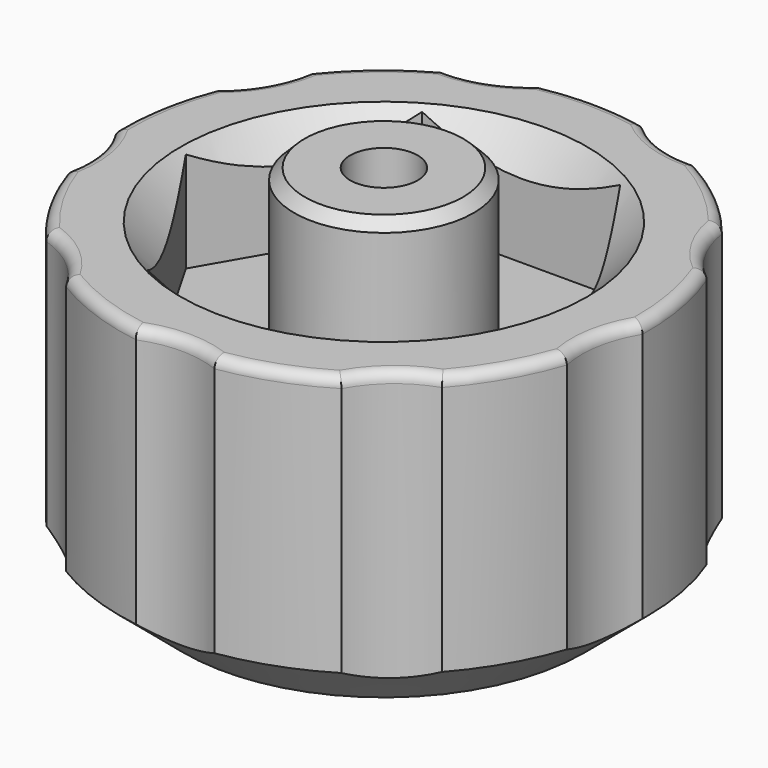
from build123d import *

# Parameters (mm, degrees)
F2_R         = 10
F3_DEPTH     = 30.001
F4_R         = 1
F5_T3_ANGLE  = 72.4183645551
F5_T6_ANGLE  = 34.3109861798
F5_T9_ANGLE  = 34.3109861798
F5_T12_ANGLE = 72.4183645551
F5_T15_ANGLE = 34.3109861798
F5_T18_ANGLE = 72.4183645551
F5_T21_ANGLE = 34.3109861799
F5_T24_ANGLE = 72.4183645551
F5_T27_ANGLE = 34.3109861798
F5_T30_ANGLE = 72.4183645551
F5_T33_ANGLE = 34.3109861799
F5_T36_ANGLE = 72.4183645551
F5_T39_ANGLE = 34.3109861799
F5_T42_ANGLE = 72.4183645551
F5_T45_ANGLE = 34.3109861799
F5_T48_ANGLE = 72.4183645551
F5_T51_ANGLE = 34.3109861798
F5_T54_ANGLE = 72.4183645551
F6_R         = 8.5
F7_DEPTH     = 10


# Not quite as in the source:
# - a fillet or chamfer that OpenCascade refuses, or shapes differently, is made with other operations: its cross-section is extruded or revolved along the edge and cut away or added


with BuildPart() as f1:
    # F0 (on Front) → F1 (revolve)
    with BuildSketch(Plane.XZ):
        Polygon((8, 8), (8.6999093082, 0), (18.6999093082, 0), (25, 5.2864037759), (25, 30), (19.25, 30), (16.25, 27), (16.25, 20), (8.5, 20), (8.5, 33.5), (7.5, 34.5), (3.2, 34.5), (3.2, 8), align=None)
    revolve(axis=Axis((0, 0, 15.2192509614), (0, 0, 1)))

    # F2 (on face) → F3 (cut, through all)
    with BuildSketch(Plane.XY.offset(30)):
        with Locations((11.6286848731, 31.9495491067)):
            Circle(F2_R)
        with Locations((-11.6286848731, 31.9495491067)):
            Circle(F2_R)
        with Locations((-29.4448637287, 17)):
            Circle(F2_R)
        with Locations((-33.4834636024, -5.9040380407)):
            Circle(F2_R)
        with Locations((-21.8547787293, -26.045511066)):
            Circle(F2_R)
        with Locations((0, -34)):
            Circle(F2_R)
        with Locations((21.8547787293, -26.045511066)):
            Circle(F2_R)
        with Locations((33.4834636024, -5.9040380407)):
            Circle(F2_R)
        with Locations((29.4448637287, 17)):
            Circle(F2_R)
    extrude(amount=-F3_DEPTH, mode=Mode.SUBTRACT)

    # F4
    f4_edges = [f1.edges().sort_by_distance(p)[0] for p in [
        (-8.699909, 0, 0),
        (-18.699909, 0, 0),
    ]]
    fillet(f4_edges, radius=F4_R)

    # F5: fillet of radius 1 on 18 edges, made by hand


with BuildPart() as f5_tool1:
    # F5_s2 → F5_t3 (revolve)
    with BuildSketch(Plane(origin=(4.7878159953, -19.5059893322, 0), x_dir=(0, 0, 1), z_dir=(0.2383778196, -0.971172495, 0))):
        with BuildLine():
            ThreePointArc((29, 17.4334321252), (29.7071067812, 17.1405389064), (30, 16.4334321252))
            Line((30, 16.4334321252), (30, 17.4334321252))
            Line((30, 17.4334321252), (29, 17.4334321252))
        make_face()
    revolve(axis=Axis((-21.8547787293, -26.045511066, 30), (0, 0, 1)), revolution_arc=F5_T3_ANGLE)


with BuildPart() as f5_tool4:
    # F5_s5 → F5_t6 (revolve)
    with BuildSketch(Plane(origin=(0, 0, 0), x_dir=(0, 0, 1), z_dir=(-0.7969993255, 0.6039801944, 0))):
        with BuildLine():
            ThreePointArc((29, -25), (29.7071067812, -24.7071067812), (30, -24))
            Line((30, -24), (30, -25))
            Line((30, -25), (29, -25))
        make_face()
    revolve(axis=Axis((0, 0, 30), (0, 0, 1)), revolution_arc=F5_T6_ANGLE)


with BuildPart() as f5_tool7:
    # F5_s8 → F5_t9 (revolve)
    with BuildSketch(Plane(origin=(0, 0, 0), x_dir=(0, 0, 1), z_dir=(-0.222305919, 0.974976963, 0))):
        with BuildLine():
            ThreePointArc((29, -25), (29.7071067812, -24.7071067812), (30, -24))
            Line((30, -24), (30, -25))
            Line((30, -25), (29, -25))
        make_face()
    revolve(axis=Axis((0, 0, 30), (0, 0, 1)), revolution_arc=F5_T9_ANGLE)


with BuildPart() as f5_tool10:
    # F5_s11 → F5_t12 (revolve)
    with BuildSketch(Plane(origin=(-8.8705284196, -18.0200035347, 0), x_dir=(0, 0, 1), z_dir=(-0.4416496426, -0.897187602, 0))):
        with BuildLine():
            ThreePointArc((29, 17.4334321252), (29.7071067812, 17.1405389064), (30, 16.4334321252))
            Line((30, 16.4334321252), (30, 17.4334321252))
            Line((30, 17.4334321252), (29, 17.4334321252))
        make_face()
    revolve(axis=Axis((-33.4834636024, -5.9040380407, 30), (0, 0, 1)), revolution_arc=F5_T12_ANGLE)


with BuildPart() as f5_tool13:
    # F5_s14 → F5_t15 (revolve)
    with BuildSketch(Plane(origin=(0, 0, 0), x_dir=(0, 0, 1), z_dir=(0.4564068976, 0.889771175, 0))):
        with BuildLine():
            ThreePointArc((29, -25), (29.7071067812, -24.7071067812), (30, -24))
            Line((30, -24), (30, -25))
            Line((30, -25), (29, -25))
        make_face()
    revolve(axis=Axis((0, 0, 30), (0, 0, 1)), revolution_arc=F5_T15_ANGLE)


with BuildPart() as f5_tool16:
    # F5_s17 → F5_t18 (revolve)
    with BuildSketch(Plane(origin=(-18.378254002, -8.1022578133, 0), x_dir=(0, 0, 1), z_dir=(-0.9150243287, -0.4033986588, 0))):
        with BuildLine():
            ThreePointArc((29, 17.4334321252), (29.7071067812, 17.1405389064), (30, 16.4334321252))
            Line((30, 16.4334321252), (30, 17.4334321252))
            Line((30, 17.4334321252), (29, 17.4334321252))
        make_face()
    revolve(axis=Axis((-29.4448637287, 17, 30), (0, 0, 1)), revolution_arc=F5_T18_ANGLE)


with BuildPart() as f5_tool19:
    # F5_s20 → F5_t21 (revolve)
    with BuildSketch(Plane(origin=(0, 0, 0), x_dir=(0, 0, 1), z_dir=(0.9215618544, 0.3882315655, 0))):
        with BuildLine():
            ThreePointArc((29, -25), (29.7071067812, -24.7071067812), (30, -24))
            Line((30, -24), (30, -25))
            Line((30, -25), (29, -25))
        make_face()
    revolve(axis=Axis((0, 0, 30), (0, 0, 1)), revolution_arc=F5_T21_ANGLE)


with BuildPart() as f5_tool22:
    # F5_s23 → F5_t24 (revolve)
    with BuildSketch(Plane(origin=(-19.2865902853, 5.6066243856, 0), x_dir=(0, 0, 1), z_dir=(-0.960248962, 0.2791450001, 0))):
        with BuildLine():
            ThreePointArc((29, 17.4334321252), (29.7071067812, 17.1405389064), (30, 16.4334321252))
            Line((30, 16.4334321252), (30, 17.4334321252))
            Line((30, 17.4334321252), (29, 17.4334321252))
        make_face()
    revolve(axis=Axis((-11.6286848731, 31.9495491067, 30), (0, 0, 1)), revolution_arc=F5_T24_ANGLE)


with BuildPart() as f5_tool25:
    # F5_s26 → F5_t27 (revolve)
    with BuildSketch(Plane(origin=(0, 0, 0), x_dir=(0, 0, 1), z_dir=(0.9555077776, -0.2949659082, 0))):
        with BuildLine():
            ThreePointArc((29, -25), (29.7071067812, -24.7071067812), (30, -24))
            Line((30, -24), (30, -25))
            Line((30, -25), (29, -25))
        make_face()
    revolve(axis=Axis((0, 0, 30), (0, 0, 1)), revolution_arc=F5_T27_ANGLE)


with BuildPart() as f5_tool28:
    # F5_s29 → F5_t30 (revolve)
    with BuildSketch(Plane(origin=(-11.1705166275, 16.6921047237, 0), x_dir=(0, 0, 1), z_dir=(-0.556162434, 0.8310736111, 0))):
        with BuildLine():
            ThreePointArc((29, 17.4334321252), (29.7071067812, 17.1405389064), (30, 16.4334321252))
            Line((30, 16.4334321252), (30, 17.4334321252))
            Line((30, 17.4334321252), (29, 17.4334321252))
        make_face()
    revolve(axis=Axis((11.6286848731, 31.9495491067, 30), (0, 0, 1)), revolution_arc=F5_T30_ANGLE)


with BuildPart() as f5_tool31:
    # F5_s32 → F5_t33 (revolve)
    with BuildSketch(Plane(origin=(0, 0, 0), x_dir=(0, 0, 1), z_dir=(0.5423609923, -0.8401455553, 0))):
        with BuildLine():
            ThreePointArc((29, -25), (29.7071067812, -24.7071067812), (30, -24))
            Line((30, -24), (30, -25))
            Line((30, -25), (29, -25))
        make_face()
    revolve(axis=Axis((0, 0, 30), (0, 0, 1)), revolution_arc=F5_T33_ANGLE)


with BuildPart() as f5_tool34:
    # F5_s35 → F5_t36 (revolve)
    with BuildSketch(Plane(origin=(2.1723659067, 19.9671637495, 0), x_dir=(0, 0, 1), z_dir=(0.1081586779, 0.9941336431, 0))):
        with BuildLine():
            ThreePointArc((29, 17.4334321252), (29.7071067812, 17.1405389064), (30, 16.4334321252))
            Line((30, 16.4334321252), (30, 17.4334321252))
            Line((30, 17.4334321252), (29, 17.4334321252))
        make_face()
    revolve(axis=Axis((29.4448637287, 17, 30), (0, 0, 1)), revolution_arc=F5_T36_ANGLE)


with BuildPart() as f5_tool37:
    # F5_s38 → F5_t39 (revolve)
    with BuildSketch(Plane(origin=(0, 0, 0), x_dir=(0, 0, 1), z_dir=(-0.4564068976, 0.889771175, 0))):
        with BuildLine():
            ThreePointArc((29, 25), (29.7071067812, 24.7071067812), (30, 24))
            Line((30, 24), (30, 25))
            Line((30, 25), (29, 25))
        make_face()
    revolve(axis=Axis((0, 0, 30), (0, 0, -1)), revolution_arc=F5_T39_ANGLE)


with BuildPart() as f5_tool40:
    # F5_s41 → F5_t42 (revolve)
    with BuildSketch(Plane(origin=(14.49877429, 13.8993649467, 0), x_dir=(0, 0, 1), z_dir=(0.7218711424, 0.692027495, 0))):
        with BuildLine():
            ThreePointArc((29, 17.4334321252), (29.7071067812, 17.1405389064), (30, 16.4334321252))
            Line((30, 16.4334321252), (30, 17.4334321252))
            Line((30, 17.4334321252), (29, 17.4334321252))
        make_face()
    revolve(axis=Axis((33.4834636024, -5.9040380407, 30), (0, 0, 1)), revolution_arc=F5_T42_ANGLE)


with BuildPart() as f5_tool43:
    # F5_s44 → F5_t45 (revolve)
    with BuildSketch(Plane(origin=(0, 0, 0), x_dir=(0, 0, 1), z_dir=(-0.7332018585, -0.6800110548, 0))):
        with BuildLine():
            ThreePointArc((29, -25), (29.7071067812, -24.7071067812), (30, -24))
            Line((30, -24), (30, -25))
            Line((30, -25), (29, -25))
        make_face()
    revolve(axis=Axis((0, 0, 30), (0, 0, 1)), revolution_arc=F5_T45_ANGLE)


with BuildPart() as f5_tool46:
    # F5_s47 → F5_t48 (revolve)
    with BuildSketch(Plane(origin=(20.0410450471, 1.327898811, 0), x_dir=(0, 0, 1), z_dir=(0.9978120766, 0.0661139909, 0))):
        with BuildLine():
            ThreePointArc((29, 17.4334321252), (29.7071067812, 17.1405389064), (30, 16.4334321252))
            Line((30, 16.4334321252), (30, 17.4334321252))
            Line((30, 17.4334321252), (29, 17.4334321252))
        make_face()
    revolve(axis=Axis((21.8547787293, -26.045511066, 30), (0, 0, 1)), revolution_arc=F5_T48_ANGLE)


with BuildPart() as f5_tool49:
    # F5_s50 → F5_t51 (revolve)
    with BuildSketch(Plane(origin=(0, 0, 0), x_dir=(0, 0, 1), z_dir=(-0.9987678899, -0.0496256197, 0))):
        with BuildLine():
            ThreePointArc((29, -25), (29.7071067812, -24.7071067812), (30, -24))
            Line((30, -24), (30, -25))
            Line((30, -25), (29, -25))
        make_face()
    revolve(axis=Axis((0, 0, 30), (0, 0, 1)), revolution_arc=F5_T51_ANGLE)


with BuildPart() as f5_tool52:
    # F5_s53 → F5_t54 (revolve)
    with BuildSketch(Plane(origin=(16.2058880953, -11.8649059363, 0), x_dir=(0, 0, 1), z_dir=(0.8068656507, -0.5907349843, 0))):
        with BuildLine():
            ThreePointArc((29, 17.4334321252), (29.7071067812, 17.1405389064), (30, 16.4334321252))
            Line((30, 16.4334321252), (30, 17.4334321252))
            Line((30, 17.4334321252), (29, 17.4334321252))
        make_face()
    revolve(axis=Axis((0, -34, 30), (0, 0, 1)), revolution_arc=F5_T54_ANGLE)


with BuildPart() as f1_1:
    add(f1.part)

    # F5_t55: cut F5_tool1, F5_tool4, F5_tool7, F5_tool10, F5_tool13, F5_tool16, F5_tool19, F5_tool22, F5_tool25, F5_tool28, F5_tool31, F5_tool34, F5_tool37, F5_tool40, F5_tool43, F5_tool46, F5_tool49, F5_tool52
    add([f5_tool1.part, f5_tool4.part, f5_tool7.part, f5_tool10.part, f5_tool13.part, f5_tool16.part, f5_tool19.part, f5_tool22.part, f5_tool25.part, f5_tool28.part, f5_tool31.part, f5_tool34.part, f5_tool37.part, f5_tool40.part, f5_tool43.part, f5_tool46.part, f5_tool49.part, f5_tool52.part], mode=Mode.SUBTRACT)

    # F6 (on face) → F7 (cut, through all)
    with BuildSketch(Plane.XY.offset(30)):
        Polygon((9.3819418743, 16.25), (-9.3819418743, 16.25), (-18.7638837487, 0), (-9.3819418743, -16.25), (9.3819418743, -16.25), (18.7638837487, 0), align=None)
        Circle(F6_R, mode=Mode.SUBTRACT)
    extrude(amount=-F7_DEPTH, mode=Mode.SUBTRACT)


solid = f1_1.part
